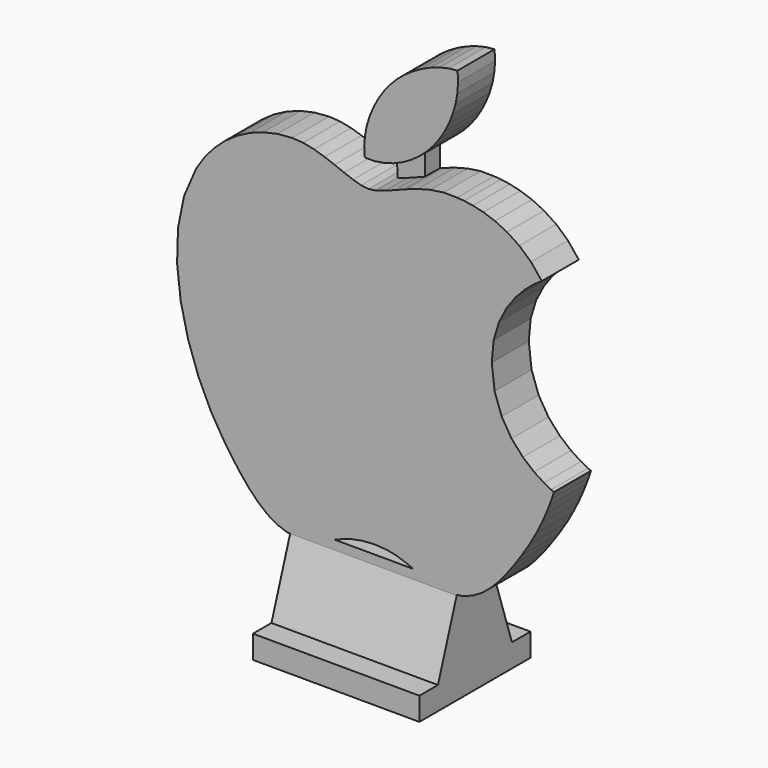
from build123d import *

# Parameters (mm, degrees)
F1_DEPTH = 2
F2_DEPTH = 5
F5_DEPTH = 18


# Not quite as in the source:
# - ends of sketch curves that miss each other by under 0.0002 mm in the source are joined


with BuildPart() as f1:
    # F0 (on Front) → F1 (new body)
    with BuildSketch(Plane.XZ):
        Polygon((13.9564371829, -4.1763302545), (13.6505568212, -1.5672102939), (13.8570021684, 0.6546701968), (14.4386421574, 2.572777133), (15.2749946567, 4.1916956816), (16.2455787436, 5.5160118155), (17.2299147044, 6.5503102987), (18.1075224224, 7.29917791), (18.7579217808, 7.7671990103), (19.0606326631, 7.9589595725), (17.8894090385, 9.4061765559), (16.6182390109, 10.5424416074), (15.3009021796, 11.4051715106), (13.991178144, 12.0317814369), (12.7428465032, 12.45968817), (11.6096864535, 12.7263080903), (10.6454779973, 12.8690567726), (9.9040003307, 12.9253510002), (8.4536993007, 12.9401075165), (7.0393171578, 12.7333035124), (5.6789414949, 12.3726223866), (4.3906586959, 11.9257463288), (4.0349177671, 11.7875631309), (3.1925567568, 11.4603583345), (2.1027220613, 11.0441405935), (1.1392422025, 10.7447756984), (1.0630562956, 10.7340944764), (0.3202043703, 10.6299470477), (-0.4697068924, 10.7259466125), (-1.3499739104, 10.9785104051), (-2.3101170508, 11.3344870803), (-3.3396570834, 11.740725293), (-4.428114778, 12.144073295), (-5.5650109045, 12.4913797411), (-6.7398666357, 12.7294928833), (-7.9422027416, 12.8052613763), (-9.5179845331, 12.6738502829), (-11.0461403111, 12.3335924529), (-12.5103628719, 11.7956320422), (-13.8943458175, 11.0711148186), (-15.1817823473, 10.171185744), (-16.3563656605, 9.1069897803), (-17.4017889563, 7.8896718894), (-18.3017458369, 6.530377436), (-19.6083064378, 3.5020943147), (-20.2715944756, 0.231420362), (-20.3699313552, -3.1782734497), (-19.9816400935, -6.6236177604), (-19.1850429015, -10.0012415978), (-18.0584619901, -13.2077743927), (-16.6802199733, -16.139845979), (-15.1286390619, -18.6940861905), (-14.3199712507, -19.8437521157), (-13.468975877, -20.9834397215), (-12.5711806097, -22.0670519206), (-11.6221131177, -23.0484932379), (-10.617301876, -23.881667795), (-9.5522737476, -24.5204789077), (-8.4225572075, -24.9188306978), (-6.2785486616, -24.924760094), (-6.1172446521, -24.9066919741), (-5.1420524281, -24.6576772732), (-4.2440729965, -24.3272277028), (-3.3692761011, -23.9589889904), (-2.4636318887, -23.5966060577), (-1.4731105063, -23.2837238261), (-0.3436821007, -23.0639884263), (0.9786835843, -22.9810443767), (2.2966708338, -23.0689926979), (3.415326636, -23.3003344778), (4.3935835633, -23.6263149411), (5.2903729793, -23.9981789094), (6.1646270535, -24.3671716073), (7.0752771494, -24.6845382594), (8.0812554366, -24.9015236875), (9.211135995, -24.9675978327), (9.2543495324, -24.9677173425), (10.4646266505, -24.8118393056), (11.5846824237, -24.4101431404), (12.6153226062, -23.7990147009), (13.5702096091, -23.0131824556), (14.4630054406, -22.087375679), (15.3073721089, -21.0563232426), (16.1169720251, -19.9547548237), (16.9054676003, -18.817399697), (17.7450979821, -17.5059903767), (18.4573257656, -16.2416880249), (19.0477701778, -15.0611340813), (19.522050849, -14.0009703886), (19.8857874094, -13.0978387898), (20.1446002953, -12.3883807244), (20.3041087338, -11.9092380354), (20.3699323552, -11.6970525654), (20.0632597243, -11.5632690975), (19.2992902384, -11.1660557409), (18.2304933913, -10.4753497913), (17.0093394832, -9.461087335), (15.7882988139, -8.0932056676), (14.7198412805, -6.3416408756), align=None)
        Polygon((3.1925567568, 11.4603583345), (4.0349177671, 11.7875631309), (4.0349177671, 14.3890940084), (3.0470887296, 13.9600045134), (2.0233786856, 13.6566557055), (0.9776241359, 13.4953402808), (1.0630562956, 10.7340944764), (1.1392422025, 10.7447756984), (2.1027220613, 11.0441405935), align=None)
        Polygon((3.0470887296, 13.9600045134), (4.0349177671, 14.3890940084), (4.9730284914, 14.9276318971), (5.8475844015, 15.5593258862), (6.6447481909, 16.2678824734), (7.3506829556, 17.0370097684), (7.9776442852, 17.8678175927), (8.5401819643, 18.7665723681), (9.0274431955, 19.7233570289), (9.4285759872, 20.7282545094), (9.7327275419, 21.7713473411), (9.9290458681, 22.8427184583), (10.0066785712, 23.9324507955), (9.9547732566, 25.030626884), (8.9884152767, 24.9252998211), (7.9933494289, 24.6925222045), (6.9902835166, 24.3433068169), (5.9999257462, 23.888667247), (5.0429839212, 23.3396154714), (4.1401666508, 22.7071646759), (3.3121821416, 22.0023272402), (2.5797377939, 21.2361167529), (1.9848069462, 20.4835481245), (1.4275088821, 19.6401188001), (0.9265880606, 18.7204873704), (0.5007873288, 17.7393128294), (0.1688511456, 16.7112529619), (-0.0504776421, 15.6509671648), (-0.1384553812, 14.5731136257), (-0.0763380157, 13.4923513387), (0.9776241359, 13.4953402808), (2.0233786856, 13.6566557055), align=None)
    extrude(amount=F1_DEPTH)

    # F0 (on Front) → F2 (join)
    with BuildSketch(Plane.XZ):
        Polygon((13.9564371829, -4.1763302545), (13.6505568212, -1.5672102939), (13.8570021684, 0.6546701968), (14.4386421574, 2.572777133), (15.2749946567, 4.1916956816), (16.2455787436, 5.5160118155), (17.2299147044, 6.5503102987), (18.1075224224, 7.29917791), (18.7579217808, 7.7671990103), (19.0606326631, 7.9589595725), (17.8894090385, 9.4061765559), (16.6182390109, 10.5424416074), (15.3009021796, 11.4051715106), (13.991178144, 12.0317814369), (12.7428465032, 12.45968817), (11.6096864535, 12.7263080903), (10.6454779973, 12.8690567726), (9.9040003307, 12.9253510002), (8.4536993007, 12.9401075165), (7.0393171578, 12.7333035124), (5.6789414949, 12.3726223866), (4.3906586959, 11.9257463288), (4.0349177671, 11.7875631309), (3.1925567568, 11.4603583345), (2.1027220613, 11.0441405935), (1.1392422025, 10.7447756984), (1.0630562956, 10.7340944764), (0.3202043703, 10.6299470477), (-0.4697068924, 10.7259466125), (-1.3499739104, 10.9785104051), (-2.3101170508, 11.3344870803), (-3.3396570834, 11.740725293), (-4.428114778, 12.144073295), (-5.5650109045, 12.4913797411), (-6.7398666357, 12.7294928833), (-7.9422027416, 12.8052613763), (-9.5179845331, 12.6738502829), (-11.0461403111, 12.3335924529), (-12.5103628719, 11.7956320422), (-13.8943458175, 11.0711148186), (-15.1817823473, 10.171185744), (-16.3563656605, 9.1069897803), (-17.4017889563, 7.8896718894), (-18.3017458369, 6.530377436), (-19.6083064378, 3.5020943147), (-20.2715944756, 0.231420362), (-20.3699313552, -3.1782734497), (-19.9816400935, -6.6236177604), (-19.1850429015, -10.0012415978), (-18.0584619901, -13.2077743927), (-16.6802199733, -16.139845979), (-15.1286390619, -18.6940861905), (-14.3199712507, -19.8437521157), (-13.468975877, -20.9834397215), (-12.5711806097, -22.0670519206), (-11.6221131177, -23.0484932379), (-10.617301876, -23.881667795), (-9.5522737476, -24.5204789077), (-8.4225572075, -24.9188306978), (-6.2785486616, -24.924760094), (-6.1172446521, -24.9066919741), (-5.1420524281, -24.6576772732), (-4.2440729965, -24.3272277028), (-3.3692761011, -23.9589889904), (-2.4636318887, -23.5966060577), (-1.4731105063, -23.2837238261), (-0.3436821007, -23.0639884263), (0.9786835843, -22.9810443767), (2.2966708338, -23.0689926979), (3.415326636, -23.3003344778), (4.3935835633, -23.6263149411), (5.2903729793, -23.9981789094), (6.1646270535, -24.3671716073), (7.0752771494, -24.6845382594), (8.0812554366, -24.9015236875), (9.211135995, -24.9675978327), (9.2543495324, -24.9677173425), (10.4646266505, -24.8118393056), (11.5846824237, -24.4101431404), (12.6153226062, -23.7990147009), (13.5702096091, -23.0131824556), (14.4630054406, -22.087375679), (15.3073721089, -21.0563232426), (16.1169720251, -19.9547548237), (16.9054676003, -18.817399697), (17.7450979821, -17.5059903767), (18.4573257656, -16.2416880249), (19.0477701778, -15.0611340813), (19.522050849, -14.0009703886), (19.8857874094, -13.0978387898), (20.1446002953, -12.3883807244), (20.3041087338, -11.9092380354), (20.3699323552, -11.6970525654), (20.0632597243, -11.5632690975), (19.2992902384, -11.1660557409), (18.2304933913, -10.4753497913), (17.0093394832, -9.461087335), (15.7882988139, -8.0932056676), (14.7198412805, -6.3416408756), align=None)
        Polygon((3.0470887296, 13.9600045134), (4.0349177671, 14.3890940084), (4.9730284914, 14.9276318971), (5.8475844015, 15.5593258862), (6.6447481909, 16.2678824734), (7.3506829556, 17.0370097684), (7.9776442852, 17.8678175927), (8.5401819643, 18.7665723681), (9.0274431955, 19.7233570289), (9.4285759872, 20.7282545094), (9.7327275419, 21.7713473411), (9.9290458681, 22.8427184583), (10.0066785712, 23.9324507955), (9.9547732566, 25.030626884), (8.9884152767, 24.9252998211), (7.9933494289, 24.6925222045), (6.9902835166, 24.3433068169), (5.9999257462, 23.888667247), (5.0429839212, 23.3396154714), (4.1401666508, 22.7071646759), (3.3121821416, 22.0023272402), (2.5797377939, 21.2361167529), (1.9848069462, 20.4835481245), (1.4275088821, 19.6401188001), (0.9265880606, 18.7204873704), (0.5007873288, 17.7393128294), (0.1688511456, 16.7112529619), (-0.0504776421, 15.6509671648), (-0.1384553812, 14.5731136257), (-0.0763380157, 13.4923513387), (0.9776241359, 13.4953402808), (2.0233786856, 13.6566557055), align=None)
    extrude(amount=F2_DEPTH)

    # F4 (on line) → F5 (join)
    with BuildSketch(Plane(origin=(9.921820884, 0, -0.0274394463), x_dir=(0, 1, 0), z_dir=(0.9999961758, 0, -0.002765555))):
        Polygon((0, -24.9420284495), (-2.5, -24.9420284495), (-2.5, -34.9420284495), (5, -34.9420284495), (5, -32.4420284495), (2.5, -32.4420284495), align=None)
        Polygon((-2.5, -24.9420284495), (-5, -24.9420284495), (-7.5, -32.4420284495), (-10, -32.4420284495), (-10, -34.9420284495), (-2.5, -34.9420284495), align=None)
        Polygon((-5, -23.9420284495), (-5, -24.9420284495), (-2.5, -24.9420284495), (0, -24.9420284495), (0, -23.9420284495), align=None)
    extrude(amount=-F5_DEPTH)


solid = f1.part
